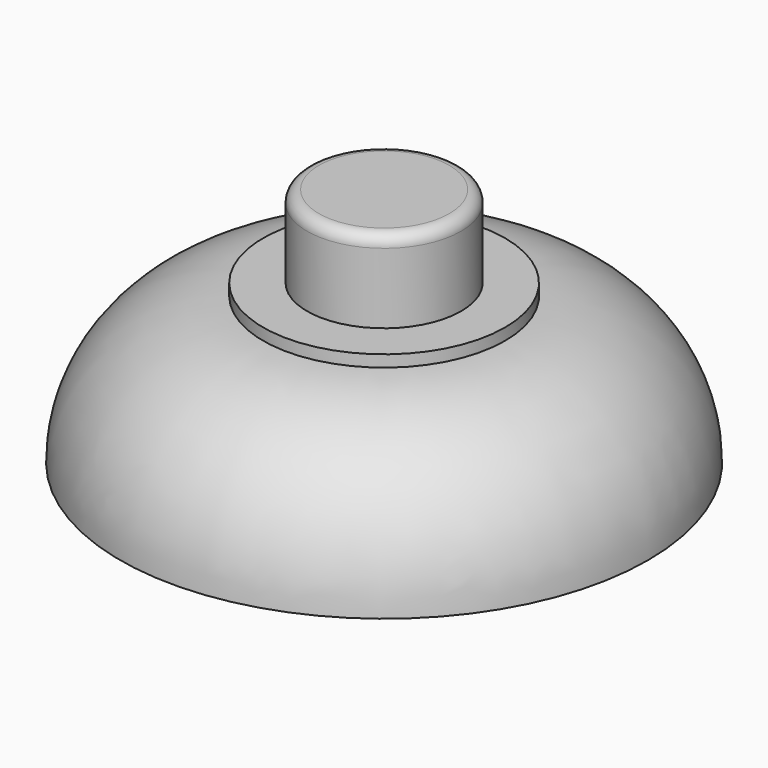
from build123d import *

# Parameters (mm, degrees)
F0_R     = 9
F0_R_2   = 4.125
F1_DEPTH = 5
F0_R_3   = 2.625
F2_DEPTH = 5.4
F3_DEPTH = 8.2
F4_R     = 7
F5_DEPTH = 4
F8_R     = 0.4


# Not quite as in the source:
# - a fillet or chamfer that OpenCascade refuses, or shapes differently, is made with other operations: its cross-section is extruded or revolved along the edge and cut away or added


with BuildPart() as f1:
    # F0 (on Top) → F1 (new body)
    with BuildSketch(Plane.XY):
        Circle(F0_R)
        Circle(F0_R_2, mode=Mode.SUBTRACT)
    extrude(amount=F1_DEPTH)

    # F0 (on Top) → F2 (join)
    with BuildSketch(Plane.XY):
        Circle(F0_R_2)
        Circle(F0_R_3, mode=Mode.SUBTRACT)
    extrude(amount=F2_DEPTH)

    # F0 (on Top) → F3 (join)
    with BuildSketch(Plane.XY):
        Circle(F0_R_3)
    extrude(amount=F3_DEPTH)

    # F4 (on face) → F5 (cut)
    with BuildSketch(Plane(origin=(0, 0, 0), x_dir=(1, 0, 0), z_dir=(0, 0, -1))):
        Circle(F4_R)
    extrude(amount=-F5_DEPTH, mode=Mode.SUBTRACT)

    # F6: fillet of radius 6 on 1 edges, made by hand

    # F6_s1 → F6_t2 (revolve)
    with BuildSketch(Plane.XZ):
        with BuildLine():
            ThreePointArc((7, 0), (4.8072473656, 2.8989794856), (1.3431457505, 4))
            Line((1.3431457505, 4), (7, 4))
            Line((7, 4), (7, 0))
        make_face()
    revolve(axis=Axis((0, 0, 4), (0, 0, -1)))

    # F7: fillet of radius 5 on 1 edges, made by hand

    # F7_s1 → F7_t2 (revolve, cut)
    with BuildSketch(Plane.XZ):
        with BuildLine():
            ThreePointArc((9, 0.0015627442), (7.5794552658, 3.4926227552), (4.125, 5))
            Line((4.125, 5), (9, 5))
            Line((9, 5), (9, 0.0015627442))
        make_face()
    revolve(axis=Axis((0, 0, 5), (0, 0, 1)), mode=Mode.SUBTRACT)

    # F8
    f8_edges = [f1.edges().sort_by_distance(p)[0] for p in [
        (-2.625, 0, 8.2),
    ]]
    fillet(f8_edges, radius=F8_R)


solid = f1.part
